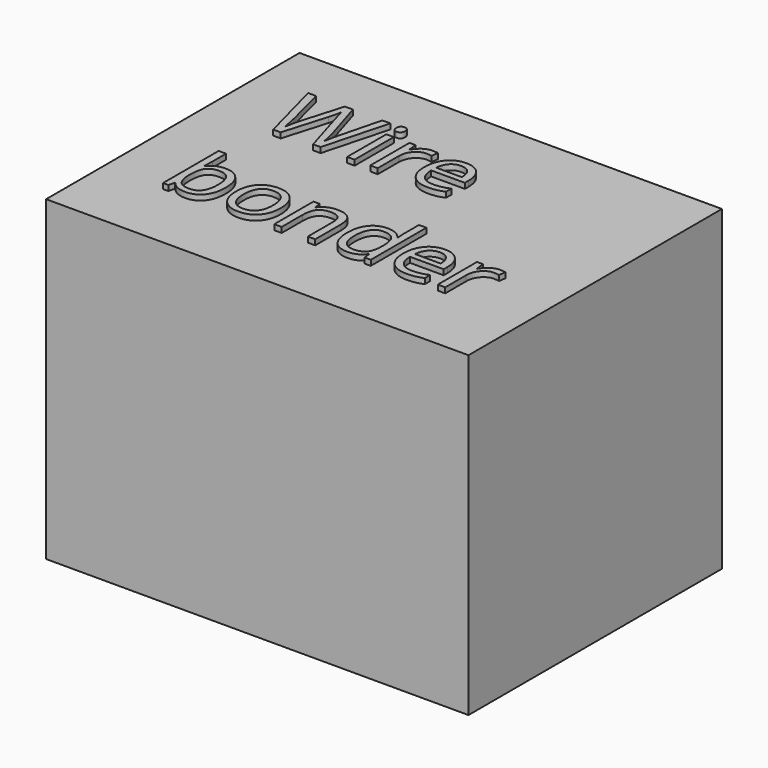
from build123d import *

# Parameters (mm, degrees)
F0_W         = 2000
F0_H         = 1500
F1_DEPTH     = 1500
F2_TEXT_SIZE = 433.0957322025
F3_DEPTH     = 25.4


# Not quite as in the source:
# - Text() gives the source's letters only with a copy of the font that has no kerning and outlines rounded to 1/6400 em; it was checked with that copy


with BuildPart() as f1:
    # F0 (on Top) → F1 (new body)
    with BuildSketch(Plane.XY):
        Rectangle(F0_W, F0_H)
    extrude(amount=F1_DEPTH)

    # F2 (on face) → F3 (join)
    with BuildSketch(Plane.XY.offset(1500)):
        with Locations((-750, 171.9021299779)):
            Text('Wire', F2_TEXT_SIZE, font='Open Sans', text_align=(TextAlign.LEFT, TextAlign.BOTTOM))
        with Locations((-750, -417.1080658175)):
            Text('bonder', F2_TEXT_SIZE, font='Open Sans', text_align=(TextAlign.LEFT, TextAlign.BOTTOM))
    extrude(amount=F3_DEPTH)


solid = f1.part
